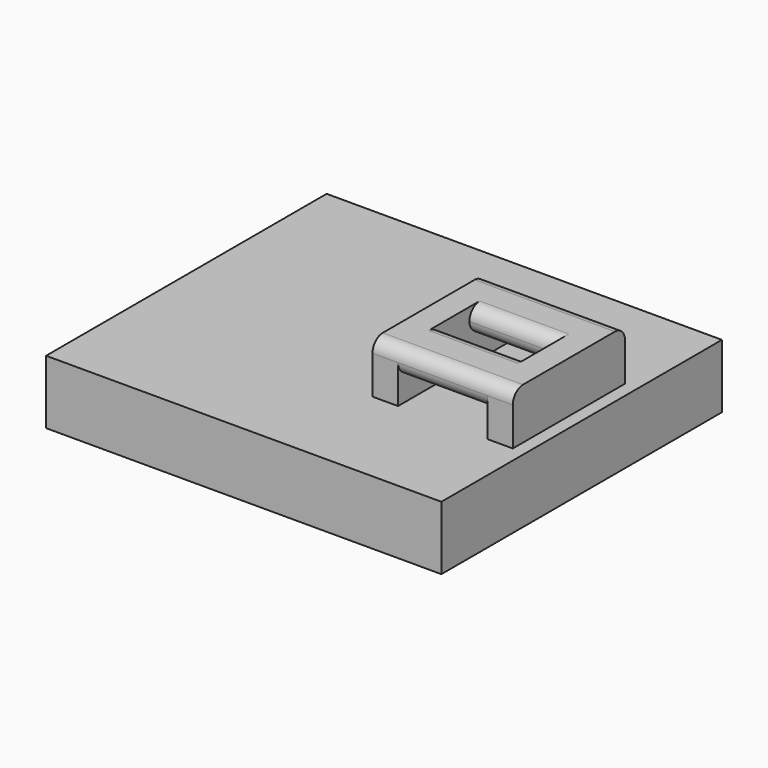
from build123d import *

# Parameters (mm, degrees)
F0_W     = 30
F0_H     = 1
F1_DEPTH = 5
F2_DEPTH = 9
F3_DEPTH = 4
F4_W     = 3.5
F4_H     = 2
F5_DEPTH = 25
F6_R     = 0.99999


# Not quite as in the source:
# - a fillet or chamfer is up to 0.001 mm smaller than in the source, because OpenCascade refuses the exact size


with BuildPart() as f1:
    # F0 (on Top) → F1 (new body)
    with BuildSketch(Plane.XY):
        with Locations((15, -0.5)):
            Rectangle(F0_W, F0_H)
        Polygon((31, 0), (30, 0), (30, -1), (30, -8.25), (30, -13.75), (30, -19.25), (30, -26.5), (30, -27.5), (31, -27.5), align=None)
        with Locations((15, -27)):
            Rectangle(F0_W, F0_H)
        Polygon((30, -1), (0, -1), (0, -13.75), (19, -13.75), (19, -8.25), (30, -8.25), align=None)
        Polygon((19, -13.75), (0, -13.75), (0, -26.5), (30, -26.5), (30, -19.25), (19, -19.25), align=None)
    extrude(amount=F1_DEPTH)

    # F0 (on Top) → F2 (join)
    with BuildSketch(Plane.XY):
        Polygon((30, -13.75), (30, -8.25), (19, -8.25), (19, -13.75), (21, -13.75), (21, -12.25), (28, -12.25), (28, -13.75), align=None)
        Polygon((21, -13.75), (19, -13.75), (19, -19.25), (30, -19.25), (30, -13.75), (28, -13.75), (28, -15.25), (21, -15.25), align=None)
    extrude(amount=F2_DEPTH)

    # F0 (on Top) → F3 (cut)
    with BuildSketch(Plane.XY):
        Polygon((30, -1), (0, -1), (0, -13.75), (19, -13.75), (19, -8.25), (30, -8.25), align=None)
        Polygon((19, -13.75), (0, -13.75), (0, -26.5), (30, -26.5), (30, -19.25), (19, -19.25), align=None)
        Polygon((21, -13.75), (19, -13.75), (19, -19.25), (30, -19.25), (30, -13.75), (28, -13.75), (28, -15.25), (21, -15.25), align=None)
        Polygon((30, -13.75), (30, -8.25), (19, -8.25), (19, -13.75), (21, -13.75), (21, -12.25), (28, -12.25), (28, -13.75), align=None)
    extrude(amount=F3_DEPTH, mode=Mode.SUBTRACT)

    # F4 (on face) → F5 (cut)
    with BuildSketch(Plane(origin=(0, -8.25, 0), x_dir=(-1, 0, 0), z_dir=(0, 1, 0))):
        with Locations((-26.25, 6)):
            Rectangle(F4_W, F4_H)
        with Locations((-22.75, 6)):
            Rectangle(F4_W, F4_H)
    extrude(amount=-F5_DEPTH, mode=Mode.SUBTRACT)

    # F6 (radius 1 in the source; OpenCascade refuses exactly that, so slightly less here)
    f6_edges = [f1.edges().sort_by_distance(p)[0] for p in [
        (24.5, -19.25, 9),
        (24.5, -12.25, 9),
        (24.5, -12.25, 7),
        (24.5, -8.25, 9),
        (24.5, -15.25, 9),
        (24.5, -15.25, 7),
        (24.5, -19.25, 7),
        (24.5, -8.25, 7),
    ]]
    fillet(f6_edges, radius=F6_R)


solid = f1.part
